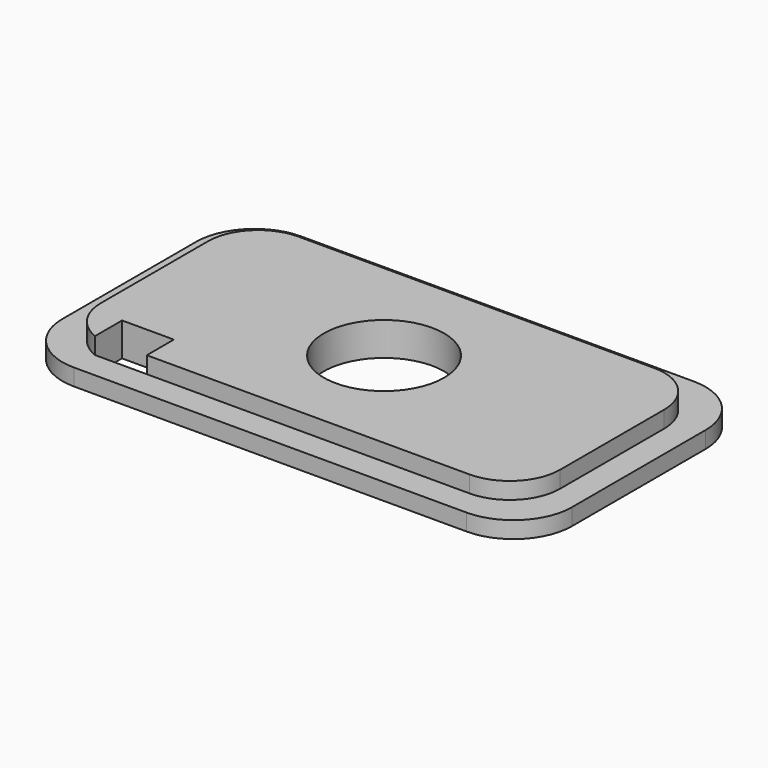
from build123d import *

# Parameters (mm, degrees)
F0_W        = 30.5
F0_H        = 17
F1_DEPTH    = 1
F2_W        = 27.3
F2_H        = 13.8
F3_DEPTH    = 1
F4_R        = 3.6
F4_W        = 3.1
F4_H        = 2.025
F5_DEPTH    = 2
F6_T1_DEPTH = 7.9496474731
F6_T3_DEPTH = 8.5
F7_R        = 3.5


# Not quite as in the source:
# - a fillet or chamfer that OpenCascade refuses, or shapes differently, is made with other operations: its cross-section is extruded or revolved along the edge and cut away or added


with BuildPart() as f1:
    # F0 (on Top) → F1 (new body)
    with BuildSketch(Plane.XY):
        Rectangle(F0_W, F0_H)
    extrude(amount=F1_DEPTH)

    # F2 (on face) → F3 (join)
    with BuildSketch(Plane.XY.offset(1)):
        Rectangle(F2_W, F2_H)
    extrude(amount=F3_DEPTH)

    # F4 (on face) → F5 (cut)
    with BuildSketch(Plane.XY.offset(2)):
        Circle(F4_R)
        with Locations((-10.228, -5.8875)):
            Rectangle(F4_W, F4_H)
    extrude(amount=-F5_DEPTH, mode=Mode.SUBTRACT)

    # F6: fillet of radius 3 on 4 edges, made by hand

    # F6_s2 → F6_t1 (cut)
    with BuildSketch(Plane.XY.offset(1)):
        with BuildLine():
            ThreePointArc((-13.65, -4.1201410108), (-13.1383729624, -5.795849816), (-11.778, -6.9))
            Line((-11.778, -6.9), (-13.65, -6.9))
            Line((-13.65, -6.9), (-13.65, -4.1201410108))
        make_face()
    extrude(amount=F6_T1_DEPTH, mode=Mode.SUBTRACT)

    # F6_s4 → F6_t3 (cut)
    with BuildSketch(Plane.XY.offset(1)):
        with BuildLine():
            ThreePointArc((13.65, -3.9), (12.7713203436, -6.0213203436), (10.65, -6.9))
            Line((10.65, -6.9), (13.65, -6.9))
            Line((13.65, -6.9), (13.65, -3.9))
        make_face()
        with BuildLine():
            ThreePointArc((-10.65, 6.9), (-12.7713203436, 6.0213203436), (-13.65, 3.9))
            Line((-13.65, 3.9), (-13.65, 6.9))
            Line((-13.65, 6.9), (-10.65, 6.9))
        make_face()
        with BuildLine():
            ThreePointArc((13.65, 3.9), (12.7713203436, 6.0213203436), (10.65, 6.9))
            Line((10.65, 6.9), (13.65, 6.9))
            Line((13.65, 6.9), (13.65, 3.9))
        make_face()
    extrude(amount=F6_T3_DEPTH, mode=Mode.SUBTRACT)

    # F7
    f7_edges = [f1.edges().sort_by_distance(p)[0] for p in [
        (15.25, 8.5, 0.5),
        (-15.25, 8.5, 0.5),
        (-15.25, -8.5, 0.5),
        (15.25, -8.5, 0.5),
    ]]
    fillet(f7_edges, radius=F7_R)


solid = f1.part
